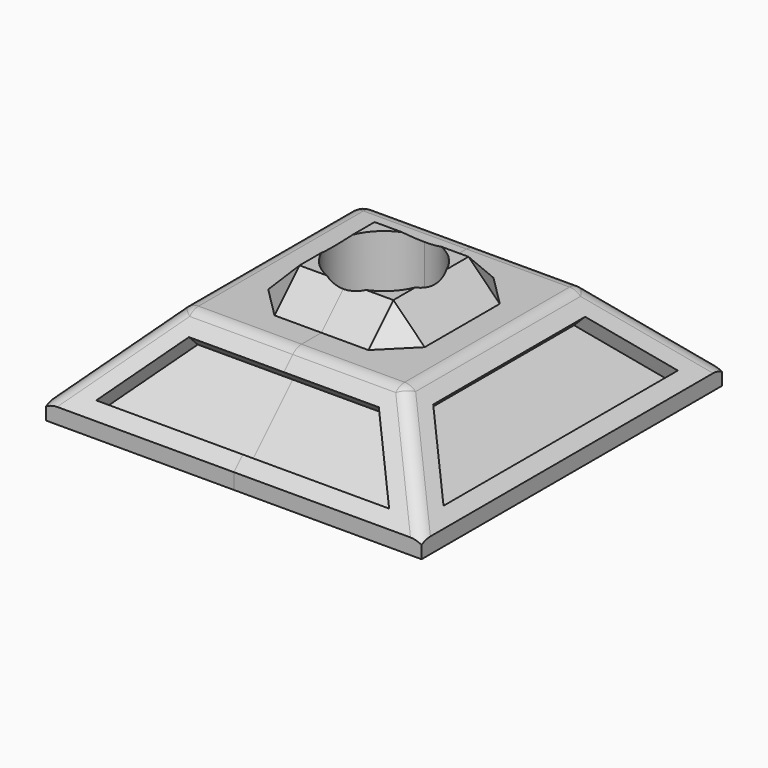
from build123d import *
from build123d import SkipClean  # not in build123d's __all__

# Parameters (mm, degrees)
F0_W      = 12
F0_H      = 12
F1_DEPTH  = 6
F2_R      = 4.7625
F3_DEPTH  = 1
F4_W      = 5
F4_H      = 5
F5_DEPTH  = 2
F6_SIZE   = 5
F7_SIZE   = 1.99999
F8_R      = 1
F10_DEPTH = 1
F12_DEPTH = 1
F13_R     = 3.25
F14_DEPTH = 7


# Not quite as in the source:
# - a fillet or chamfer is up to 0.001 mm smaller than in the source, because OpenCascade refuses the exact size


with BuildPart() as f1:
    # F0 (on Top) → F1 (new body)
    with BuildSketch(Plane.XY):
        with Locations((-6, 6)):
            Rectangle(F0_W, F0_H)
    extrude(amount=F1_DEPTH)

    # F2 (on face) → F3 (cut)
    with BuildSketch(Plane(origin=(0, 0, 0), x_dir=(1, 0, 0), z_dir=(0, 0, -1))):
        Circle(F2_R)
    extrude(amount=-F3_DEPTH, mode=Mode.SUBTRACT)

    # F4 (on face) → F5 (join)
    with BuildSketch(Plane.XY.offset(6)):
        with Locations((-2.5, 2.5)):
            Rectangle(F4_W, F4_H)
    extrude(amount=F5_DEPTH)

    # F6
    f6_edges = [f1.edges().sort_by_distance(p)[0] for p in [
        (-12, 6, 6),
        (-6, 12, 6),
    ]]
    chamfer(f6_edges, length=F6_SIZE)

    # F7 (size 2 in the source; OpenCascade refuses exactly that, so slightly less here)
    f7_edges = [f1.edges().sort_by_distance(p)[0] for p in [
        (-5, 5, 7),
        (-5, 2.5, 8),
        (-2.5, 5, 8),
    ]]
    chamfer(f7_edges, length=F7_SIZE)

    # F8
    f8_edges = [f1.edges().sort_by_distance(p)[0] for p in [
        (-7, 3.5, 6),
        (-3.5, 7, 6),
        (-9.5, 9.5, 3.5),
    ]]
    fillet(f8_edges, radius=F8_R)

    # F9 (on face) → F10 (cut)
    with BuildSketch(Plane(origin=(0, 6.5, 6.5), x_dir=(-1, 0, 0), z_dir=(0, 0.7071067812, 0.7071067812))):
        Polygon((0, -6.7781745931), (9.3610415662, -6.7781745931), (6.0681483474, -2.1213203436), (0, -2.1213203436), align=None)
    extrude(amount=-F10_DEPTH, mode=Mode.SUBTRACT)

    # F11 (on face) → F12 (cut)
    with BuildSketch(Plane(origin=(-6.5, 0, 6.5), x_dir=(0, -1, 0), z_dir=(-0.7071067812, 0, 0.7071067812))):
        Polygon((0, -6.7781745931), (0, -2.1213203436), (-6.0681483474, -2.1213203436), (-9.3610415662, -6.7781745931), align=None)
    extrude(amount=-F12_DEPTH, mode=Mode.SUBTRACT)

    # F13 (on face) → F14 (cut, through all)
    with BuildSketch(Plane.XY.offset(8)):
        Circle(F13_R)
    extrude(amount=-F14_DEPTH, mode=Mode.SUBTRACT)

    # F15: F1 across plane


with BuildPart() as f1_1:
    add(f1.part, clean=False)
    add(f1.part.mirror(Plane.XZ), clean=False)

    # F16: F1 across plane


with BuildPart() as f1_2:
    add(f1_1.part, clean=False)
    with SkipClean():  # cleaning this boolean's faces spoils the solid; the shape is the same uncleaned
        add(f1_1.part.mirror(Plane.YZ), clean=False)


solid = f1_2.part
